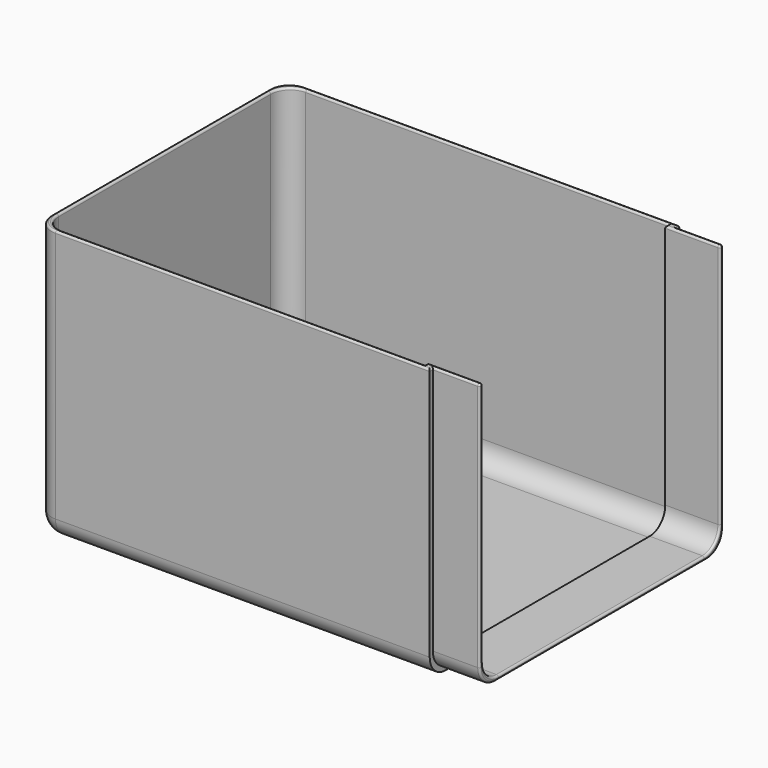
from build123d import *

# Parameters (mm, degrees)
F0_W     = 101
F0_H     = 80
F1_DEPTH = 70
F3_DEPTH = 69
F5_DEPTH = 2
F7_DEPTH = 14
F8_R     = 5
F9_R     = 0.49999


# Not quite as in the source:
# - a fillet or chamfer is up to 0.001 mm smaller than in the source, because OpenCascade refuses the exact size


with BuildPart() as f1:
    # F0 (on Top) → F1 (new body)
    with BuildSketch(Plane.XY):
        Rectangle(F0_W, F0_H)
    extrude(amount=F1_DEPTH)

    # F2 (on face) → F3 (cut)
    with BuildSketch(Plane.XY.offset(70)):
        Polygon((48.5, 39), (-49.5, 39), (-49.5, 20.586034283), (-49.5, -39), (48.5, -39), (48.5, -30.7030728576), align=None)
    extrude(amount=-F3_DEPTH, mode=Mode.SUBTRACT)

    # F4 (on face) → F5 (cut)
    with BuildSketch(Plane.YZ.offset(50.5)):
        Polygon((38, 2), (38, 70), (-38, 70), (-38, 42.2970801592), (-38, 2), align=None)
    extrude(amount=-F5_DEPTH, mode=Mode.SUBTRACT)

    # F6 (on face) → F7 (join)
    with BuildSketch(Plane(origin=(48.5, 0, 0), x_dir=(0, -1, 0), z_dir=(-1, 0, 0))):
        Polygon((39, 1), (39, 70), (38, 70), (38, 2), (-38, 2), (-38, 70), (-39, 70), (-39, 1), align=None)
    extrude(amount=-F7_DEPTH)

    # F8
    f8_edges = [f1.edges().sort_by_distance(p)[0] for p in [
        (-0.5, 39, 1),
        (-49.5, 0, 1),
        (-0.5, -39, 1),
        (0, 40, 0),
        (-50.5, 0, 0),
        (0, -40, 0),
        (-50.5, -40, 35),
        (-50.5, 40, 35),
        (-49.5, 39, 35.5),
        (-49.5, -39, 35.5),
        (56.5, 39, 1),
        (56.5, -39, 1),
        (55.5, -38, 2),
        (55.5, 38, 2),
    ]]
    fillet(f8_edges, radius=F8_R)

    # F9 (radius 0.5 in the source; OpenCascade refuses exactly that, so slightly less here)
    f9_edges = [f1.edges().sort_by_distance(p)[0] for p in [
        (2.5, 40, 70),
        (-49.035534, 38.535534, 70),
        (50.5, 39.5, 70),
        (-50.5, 0, 70),
        (56.5, 39, 70),
        (-49.035534, -38.535534, 70),
        (62.5, 38.5, 70),
        (2.5, -40, 70),
        (55.5, 38, 70),
        (50.5, -39.5, 70),
        (48.5, 38.5, 70),
        (56.5, -39, 70),
        (2, 39, 70),
        (62.5, -38.5, 70),
        (-48.035534, 37.535534, 70),
        (55.5, -38, 70),
        (-49.5, 0, 70),
        (48.5, -38.5, 70),
        (-48.035534, -37.535534, 70),
        (2, -39, 70),
        (62.5, -39, 38),
        (62.5, -37.535534, 2.464466),
        (62.5, 0, 1),
        (62.5, -38, 38.5),
        (62.5, 37.535534, 2.464466),
        (62.5, -36.535534, 3.464466),
        (62.5, 39, 38),
        (62.5, 0, 2),
        (62.5, 36.535534, 3.464466),
        (62.5, 38, 38.5),
    ]]
    fillet(f9_edges, radius=F9_R)


solid = f1.part
